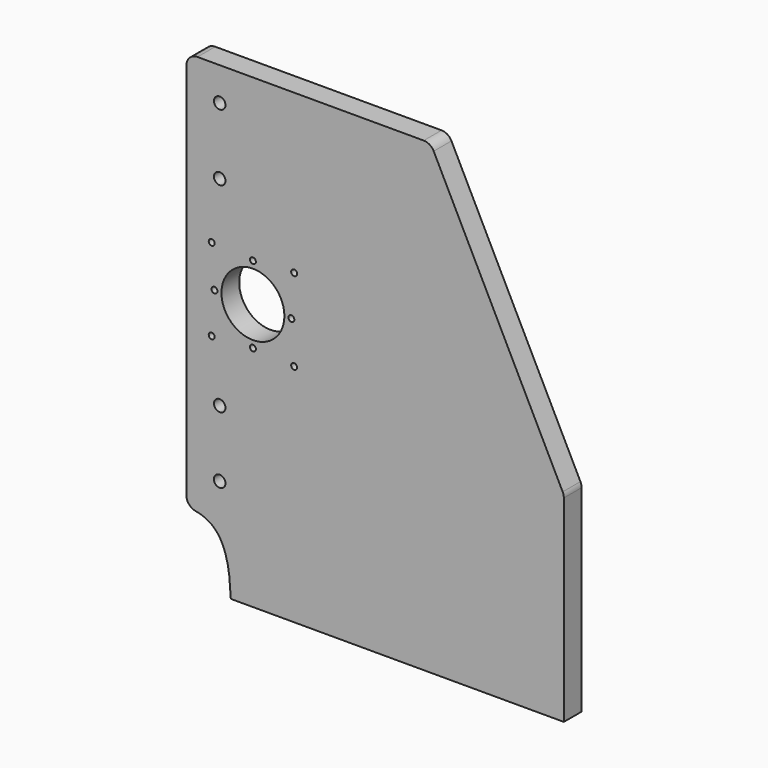
from build123d import *

# Parameters (mm, degrees)
F0_R     = 3.302
F0_R_2   = 1.7
F0_R_3   = 18
F1_DEPTH = 12.7
F2_DEPTH = 25.4
F3_R     = 6.35
F4_R     = 2.7051
F5_DEPTH = 25.4


# Not quite as in the source:
# - a feature names something its author has since deleted; it is built from what else it names


with BuildPart() as f1:
    # F0 (on Front) → F1 (new body)
    with BuildSketch(Plane.XZ):
        with BuildLine():
            Line((108.4265169831, 0.0004552842), (32.2265169831, 152.4004552842))
            Line((32.2265169831, 152.4004552842), (-107.4734830169, 152.4004552842))
            Line((-107.4734830169, 152.4004552842), (-107.4734830169, -76.1995447158))
            add(Edge.make_bspline(
                [(-82.0734830169, -114.2995447158), (-82.8863746009, -95.7832909802), (-85.4194185281, -76.1871889735), (-107.4734830169, -76.1995447158)],
                knots=[0, 0, 0, 0, 45.7905011984, 45.7905011984, 45.7905011984, 45.7905011984], degree=3))
            Line((-82.0734830169, -114.2995447158), (108.4265169831, -114.2995447158))
            Line((108.4265169831, -114.2995447158), (108.4265169831, 0.0004552842))
        make_face()
        with Locations((-88.4234830169, -57.1371889735)):
            Circle(F0_R, mode=Mode.SUBTRACT)
        with Locations((-88.4234830169, -19.0371889735)):
            Circle(F0_R, mode=Mode.SUBTRACT)
        with Locations((-92.9944827628, 14.5430932346)):
            Circle(F0_R_2, mode=Mode.SUBTRACT)
        with Locations((-69.4244827628, 16.1130932346)):
            Circle(F0_R_2, mode=Mode.SUBTRACT)
        with Locations((-45.8544827628, 14.5430932346)):
            Circle(F0_R_2, mode=Mode.SUBTRACT)
        with Locations((-91.4244827628, 38.1130932346)):
            Circle(F0_R_2, mode=Mode.SUBTRACT)
        with Locations((-69.4244827628, 38.1130932346)):
            Circle(F0_R_3, mode=Mode.SUBTRACT)
        with Locations((-92.9944827628, 61.6830932346)):
            Circle(F0_R_2, mode=Mode.SUBTRACT)
        with Locations((-69.4244827628, 60.1130932346)):
            Circle(F0_R_2, mode=Mode.SUBTRACT)
        with Locations((-47.4244827628, 38.1130932346)):
            Circle(F0_R_2, mode=Mode.SUBTRACT)
        with Locations((-45.8544827628, 61.6830932346)):
            Circle(F0_R_2, mode=Mode.SUBTRACT)
        with Locations((-88.4234830169, 95.2504552842)):
            Circle(F0_R, mode=Mode.SUBTRACT)
        with Locations((-88.4234830169, 133.3504552842)):
            Circle(F0_R, mode=Mode.SUBTRACT)
    extrude(amount=F1_DEPTH)

    # F0 (on Front) → F2 (cut)
    with BuildSketch(Plane.XZ):
        with BuildLine():
            add(Edge.make_bspline(
                [(-82.0734830169, -114.2995447158), (-82.8863746009, -95.7832909802), (-85.4194185281, -76.1871889735), (-107.4734830169, -76.1995447158)],
                knots=[0, 0, 0, 0, 45.7905011984, 45.7905011984, 45.7905011984, 45.7905011984], degree=3))
            Line((-107.4734830169, -76.1995447158), (-107.4734830169, -114.2995447158))
            Line((-107.4734830169, -114.2995447158), (-82.0734830169, -114.2995447158))
        make_face()
        with BuildLine():
            Line((108.4265169831, 0.0004552842), (32.2265169831, 152.4004552842))
            Line((32.2265169831, 152.4004552842), (-107.4734830169, 152.4004552842))
            Line((-107.4734830169, 152.4004552842), (-107.4734830169, -76.1995447158))
            add(Edge.make_bspline(
                [(-82.0734830169, -114.2995447158), (-82.8863746009, -95.7832909802), (-85.4194185281, -76.1871889735), (-107.4734830169, -76.1995447158)],
                knots=[0, 0, 0, 0, 45.7905011984, 45.7905011984, 45.7905011984, 45.7905011984], degree=3))
            Line((-82.0734830169, -114.2995447158), (108.4265169831, -114.2995447158))
            Line((108.4265169831, -114.2995447158), (108.4265169831, 0.0004552842))
        make_face()
        with Locations((-88.4234830169, -57.1371889735)):
            Circle(F0_R, mode=Mode.SUBTRACT)
        with Locations((-88.4234830169, -19.0371889735)):
            Circle(F0_R, mode=Mode.SUBTRACT)
        with Locations((-92.9944827628, 14.5430932346)):
            Circle(F0_R_2, mode=Mode.SUBTRACT)
        with Locations((-69.4244827628, 16.1130932346)):
            Circle(F0_R_2, mode=Mode.SUBTRACT)
        with Locations((-45.8544827628, 14.5430932346)):
            Circle(F0_R_2, mode=Mode.SUBTRACT)
        with Locations((-91.4244827628, 38.1130932346)):
            Circle(F0_R_2, mode=Mode.SUBTRACT)
        with Locations((-69.4244827628, 38.1130932346)):
            Circle(F0_R_3, mode=Mode.SUBTRACT)
        with Locations((-92.9944827628, 61.6830932346)):
            Circle(F0_R_2, mode=Mode.SUBTRACT)
        with Locations((-69.4244827628, 60.1130932346)):
            Circle(F0_R_2, mode=Mode.SUBTRACT)
        with Locations((-47.4244827628, 38.1130932346)):
            Circle(F0_R_2, mode=Mode.SUBTRACT)
        with Locations((-45.8544827628, 61.6830932346)):
            Circle(F0_R_2, mode=Mode.SUBTRACT)
        with Locations((-88.4234830169, 95.2504552842)):
            Circle(F0_R, mode=Mode.SUBTRACT)
        with Locations((-88.4234830169, 133.3504552842)):
            Circle(F0_R, mode=Mode.SUBTRACT)
    extrude(amount=-F2_DEPTH, mode=Mode.SUBTRACT)

    # F3
    f3_edges = [f1.edges().sort_by_distance(p)[0] for p in [
        (-107.473483, -6.35, -76.199545),
        (-107.473483, -6.35, 152.400455),
        (108.426517, -6.35, 0.000455),
        (32.226517, -6.35, 152.400455),
    ]]
    fillet(f3_edges, radius=F3_R)

    # F4 (on face) → F5 (cut)
    with BuildSketch(Plane(origin=(0, 0, -114.2995447158), x_dir=(1, 0, 0), z_dir=(0, 0, -1))):
        with Locations((-70.4482253863, 6.35)):
            Circle(F4_R)
        with Locations((-29.1732253863, 6.35)):
            Circle(F4_R)
        with Locations((12.1017746137, 6.35)):
            Circle(F4_R)
        with Locations((53.3767746137, 6.35)):
            Circle(F4_R)
        with Locations((94.6517746137, 6.35)):
            Circle(F4_R)
    extrude(amount=-F5_DEPTH, mode=Mode.SUBTRACT)


solid = f1.part
